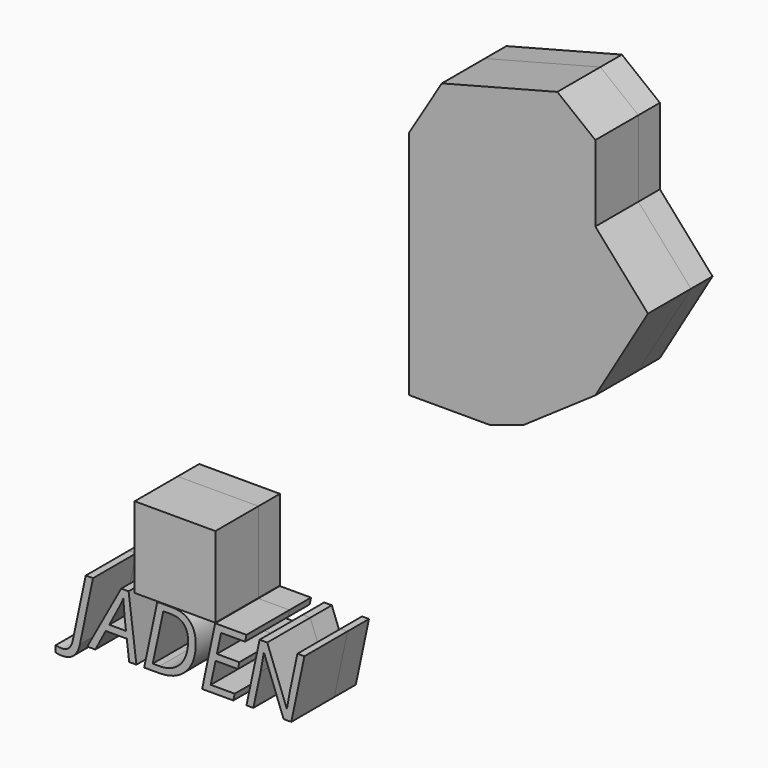
from build123d import *

# Parameters (mm, degrees)
F0_W         = 76.2
F0_H         = 76.2
F0_W_2       = 76.60394907
F0_H_2       = 84.2724889517
F0_TEXT_SIZE = 82.094131762
F1_DEPTH     = 76.2
F2_DEPTH     = 25.4


# Not quite as in the source:
# - Text() gives the source's letters only with a copy of the font that has no kerning and outlines rounded to 1/6400 em; it was checked with that copy


with BuildPart() as f1:
    # F0 (on Front) → F1 (new body)
    with BuildSketch(Plane.XZ):
        with Locations((-38.1, 38.1)):
            Rectangle(F0_W, F0_H)
        Polygon((213.7827277184, 384.5863640308), (182.7270686626, 409.1260349274), (182.7270686626, 332.9260349274), (259.3310177326, 332.9260349274), (259.3310177326, 248.6535459757), (290.3866767883, 258.593018095), (290.3866767883, 290.943801403), (290.3866767883, 342.11987257), (358.7091267109, 376.3355016708), (358.7091267109, 445.9314346313), (322.8225708008, 414.9748682976), (322.8225708008, 376.3355016708), (213.7827277184, 346.9211161137), align=None)
        Polygon((182.7270686626, 466.5710031986), (182.7270686626, 409.1260349274), (213.7827277184, 384.5863640308), (213.7827277184, 474.090307951), (213.7827277184, 517.8160667419), align=None)
        with Locations((221.0290431976, 290.7897904515)):
            Rectangle(F0_W_2, F0_H_2)
        Polygon((213.7827277184, 474.090307951), (213.7827277184, 384.5863640308), (213.7827277184, 346.9211161137), (322.8225708008, 376.3355016708), (322.8225708008, 414.9748682976), (322.8225708008, 506.375014782), (322.8225708008, 546.1730328609), (213.7827277184, 517.8160667419), align=None)
        Polygon((358.7091267109, 517.8160667419), (322.8225708008, 546.1730328609), (322.8225708008, 506.375014782), (322.8225708008, 414.9748682976), (358.7091267109, 445.9314346313), align=None)
        Polygon((290.3866767883, 290.943801403), (290.3866767883, 258.593018095), (358.7091267109, 305.6310713291), (358.7091267109, 376.3355016708), (290.3866767883, 342.11987257), align=None)
        Polygon((358.7091267109, 376.3355016708), (358.7091267109, 305.6310713291), (408.3702146969, 389.7319845336), align=None)
        Polygon((408.3702146969, 389.7319845336), (358.7091267109, 445.9314346313), (358.7091267109, 376.3355016708), align=None)
        with Locations((-138.1497532129, -59.1077748686)):
            Text('JADEN', F0_TEXT_SIZE, font='Open Sans', font_style=FontStyle.ITALIC, text_align=(TextAlign.LEFT, TextAlign.BOTTOM))
    extrude(amount=F1_DEPTH)


with BuildPart() as f2:
    # F0 (on Front) → F2 (new body)
    with BuildSketch(Plane.XZ):
        with Locations((-38.1, 38.1)):
            Rectangle(F0_W, F0_H)
        Polygon((213.7827277184, 384.5863640308), (182.7270686626, 409.1260349274), (182.7270686626, 332.9260349274), (259.3310177326, 332.9260349274), (259.3310177326, 248.6535459757), (290.3866767883, 258.593018095), (290.3866767883, 290.943801403), (290.3866767883, 342.11987257), (358.7091267109, 376.3355016708), (358.7091267109, 445.9314346313), (322.8225708008, 414.9748682976), (322.8225708008, 376.3355016708), (213.7827277184, 346.9211161137), align=None)
        Polygon((182.7270686626, 466.5710031986), (182.7270686626, 409.1260349274), (213.7827277184, 384.5863640308), (213.7827277184, 474.090307951), (213.7827277184, 517.8160667419), align=None)
        with Locations((221.0290431976, 290.7897904515)):
            Rectangle(F0_W_2, F0_H_2)
        Polygon((213.7827277184, 474.090307951), (213.7827277184, 384.5863640308), (213.7827277184, 346.9211161137), (322.8225708008, 376.3355016708), (322.8225708008, 414.9748682976), (322.8225708008, 506.375014782), (322.8225708008, 546.1730328609), (213.7827277184, 517.8160667419), align=None)
        Polygon((358.7091267109, 517.8160667419), (322.8225708008, 546.1730328609), (322.8225708008, 506.375014782), (322.8225708008, 414.9748682976), (358.7091267109, 445.9314346313), align=None)
        Polygon((290.3866767883, 290.943801403), (290.3866767883, 258.593018095), (358.7091267109, 305.6310713291), (358.7091267109, 376.3355016708), (290.3866767883, 342.11987257), align=None)
        Polygon((358.7091267109, 376.3355016708), (358.7091267109, 305.6310713291), (408.3702146969, 389.7319845336), align=None)
        Polygon((408.3702146969, 389.7319845336), (358.7091267109, 445.9314346313), (358.7091267109, 376.3355016708), align=None)
        with Locations((-138.1497532129, -59.1077748686)):
            Text('JADEN', F0_TEXT_SIZE, font='Open Sans', font_style=FontStyle.ITALIC, text_align=(TextAlign.LEFT, TextAlign.BOTTOM))
    extrude(amount=F2_DEPTH)


solid = Compound([f1.part, f2.part])
